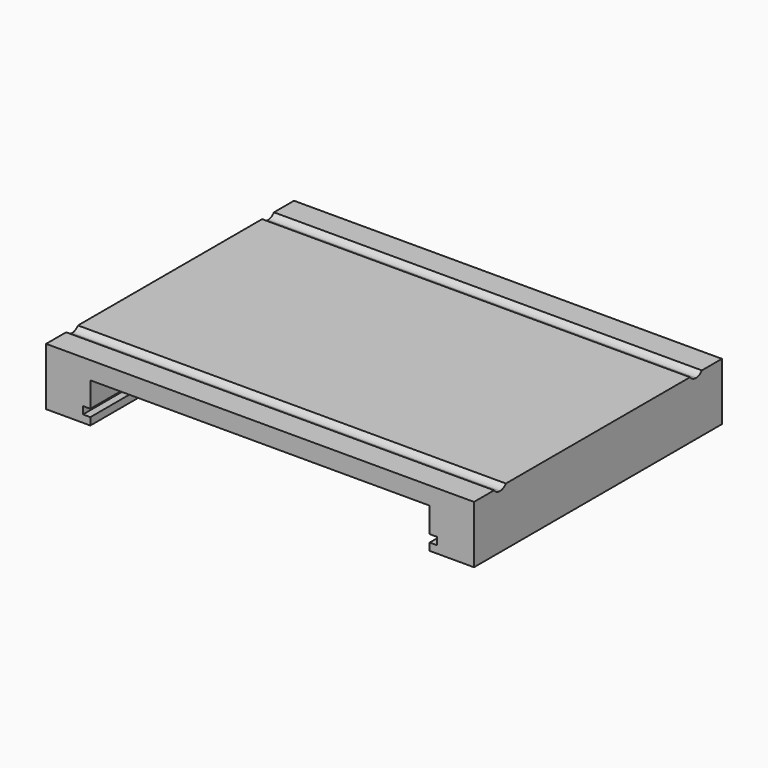
from build123d import *

# Parameters (mm, degrees)
F0_W     = 290
F0_H     = 210
F1_DEPTH = 12
F2_W     = 30
F2_H     = 210
F3_DEPTH = 27
F4_W     = 5
F4_H     = 5
F5_DEPTH = 210.001
F7_DEPTH = 290.001


# Not quite as in the source:
# - a pattern or mirror of a feature is missing from the dataset's text; its kind, count and spacing are read off the source's solid


with BuildPart() as f1:
    # F0 (on Top) → F1 (new body)
    with BuildSketch(Plane.XY):
        Rectangle(F0_W, F0_H)
    extrude(amount=-F1_DEPTH)

    # F2 (on face) → F3 (join)
    with BuildSketch(Plane(origin=(0, 0, -12), x_dir=(1, 0, 0), z_dir=(0, 0, -1))):
        with Locations((130, 0)):
            Rectangle(F2_W, F2_H)
        with Locations((-130, 0)):
            Rectangle(F2_W, F2_H)
    extrude(amount=F3_DEPTH)

    # F4 (on face) → F5 (cut, through all)
    with BuildSketch(Plane.XZ.offset(105)):
        with Locations((-117.5, -31.5)):
            Rectangle(F4_W, F4_H)
        with Locations((117.5, -31.5)):
            Rectangle(F4_W, F4_H)
    extrude(amount=-F5_DEPTH, mode=Mode.SUBTRACT)

    # F6 (on face) → F7 (cut, through all)
    with BuildSketch(Plane(origin=(-145, 0, 0), x_dir=(0, -1, 0), z_dir=(-1, 0, 0))):
        with BuildLine():
            Line((-78, 0), (-88, 0))
            ThreePointArc((-88, 0), (-85.7950849719, -1.8401699437), (-83, -2.5))
            ThreePointArc((-83, -2.5), (-80.2049150281, -1.8401699437), (-78, 0))
        make_face()
    f7 = extrude(amount=-F7_DEPTH, mode=Mode.SUBTRACT)

    # F7_copies: F7 across plane
    add(f7.mirror(Plane(origin=(0, 0, 0), x_dir=(0, 0, -1), z_dir=(0, -1, 0))), mode=Mode.SUBTRACT)


solid = f1.part
